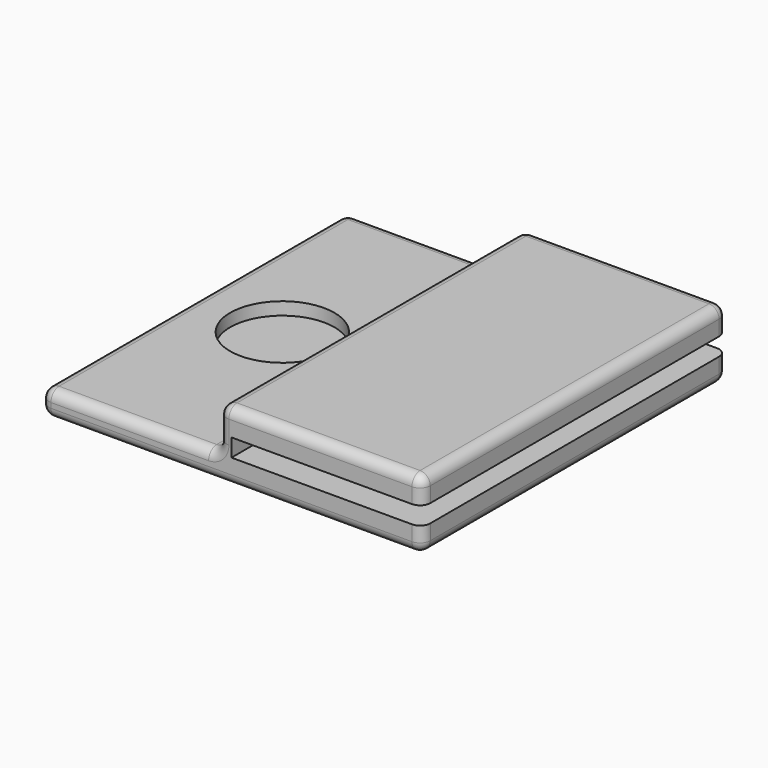
from build123d import *

# Parameters (mm, degrees)
F0_W     = 75
F0_H     = 75
F1_DEPTH = 5
F2_W     = 40
F2_H     = 75
F3_DEPTH = 8.5
F4_W     = 75
F4_H     = 3.5
F5_DEPTH = 37.5
F6_R     = 10.25
F7_DEPTH = 2.5
F8_R     = 2


with BuildPart() as f1:
    # F0 (on Top) → F1 (new body)
    with BuildSketch(Plane.XY):
        Rectangle(F0_W, F0_H)
    extrude(amount=F1_DEPTH)

    # F2 (on face) → F3 (join)
    with BuildSketch(Plane.XY.offset(5)):
        with Locations((17.5, 0)):
            Rectangle(F2_W, F2_H)
    extrude(amount=F3_DEPTH)

    # F4 (on face) → F5 (cut, through all)
    with BuildSketch(Plane.YZ.offset(37.5)):
        with Locations((0, 6.75)):
            Rectangle(F4_W, F4_H)
    extrude(amount=-F5_DEPTH, mode=Mode.SUBTRACT)

    # F6 (on face) → F7 (cut)
    with BuildSketch(Plane.XY.offset(5)):
        with Locations((-20, 0)):
            Circle(F6_R)
    extrude(amount=-F7_DEPTH, mode=Mode.SUBTRACT)

    # F8
    f8_edges = [f1.edges().sort_by_distance(p)[0] for p in [
        (17.5, 37.5, 13.5),
        (-2.5, 0, 13.5),
        (17.5, -37.5, 13.5),
        (37.5, 0, 13.5),
        (-2.5, 37.5, 9.25),
        (-2.5, -37.5, 9.25),
        (-2.5, 0, 5),
        (-37.5, 37.5, 2.5),
        (-37.5, -37.5, 2.5),
        (-37.5, 0, 0),
        (-37.5, 0, 5),
        (0, -37.5, 0),
        (37.5, 0, 0),
        (0, 37.5, 0),
        (37.5, -37.5, 11),
        (37.5, -37.5, 2.5),
        (37.5, 37.5, 11),
        (37.5, 37.5, 2.5),
        (-20, -37.5, 5),
        (-20, 37.5, 5),
    ]]
    fillet(f8_edges, radius=F8_R)


solid = f1.part
